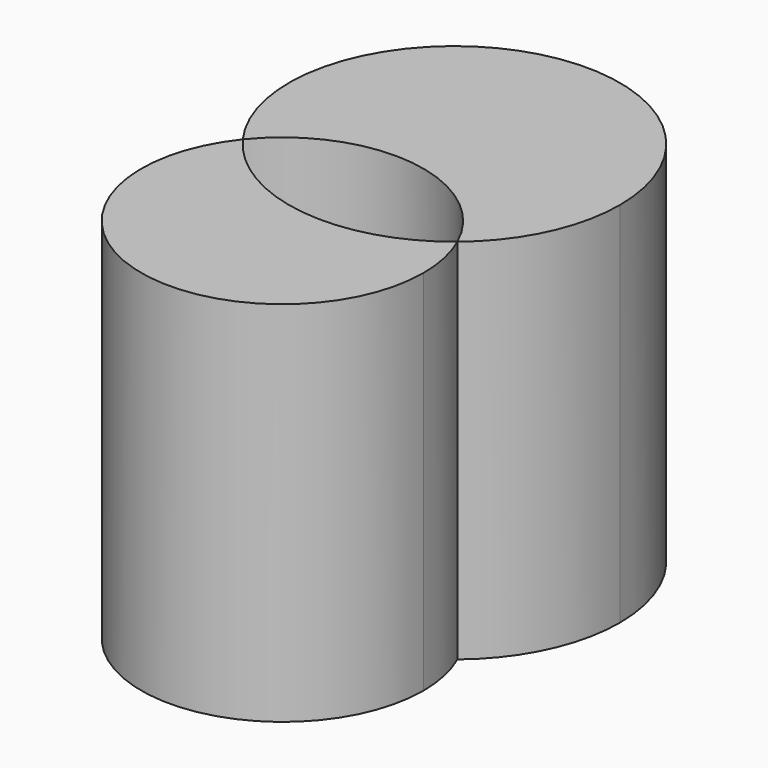
from build123d import *

# Parameters (mm, degrees)
F1_DEPTH = 76.2


with BuildPart() as f1:
    # F0 (on Top) → F1 (new body)
    with BuildSketch(Plane.XY):
        with BuildLine():
            ThreePointArc((1.8643373855, 18.6946746403), (11.0789540131, 30.5294595365), (14.3597911671, 45.1652854681))
            ThreePointArc((14.3597911671, 45.1652854681), (-30.5176686365, 77.7738686127), (-47.6673005986, 25.0178621615))
            ThreePointArc((-47.6673005986, 25.0178621615), (-21.1269727644, 35.7565883383), (1.8643373855, 18.6946746403))
        make_face()
    extrude(amount=F1_DEPTH)


with BuildPart() as f1b:
    # F0 (on Top) → F1, piece 2 (new body)
    with BuildSketch(Plane.XY):
        with BuildLine():
            ThreePointArc((1.8643373855, 18.6946746403), (-24.2675193626, 11.1556387927), (-47.6673005986, 25.0178621615))
            ThreePointArc((-47.6673005986, 25.0178621615), (-34.5135824843, -20.8544377569), (4.4172127574, 6.7441379651))
            ThreePointArc((4.4172127574, 6.7441379651), (3.7718744023, 12.854221833), (1.8643373855, 18.6946746403))
        make_face()
    extrude(amount=F1_DEPTH)


solid = Compound([f1.part, f1b.part])
